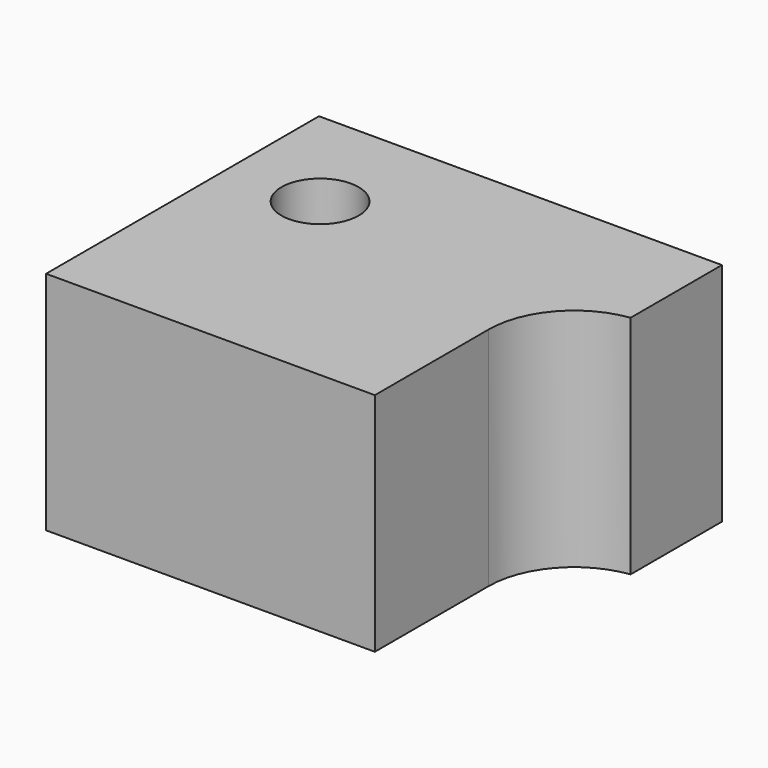
from build123d import *

# Parameters (mm, degrees)
F0_W        = 909.2783331871
F0_H        = 769.7594761848
F0_R        = 87.1640503321
F1_DEPTH    = 509.82533
F2_W        = 512.1824108064
F2_H        = 509.82533
F3_DEPTH    = 167.38894
F4_T1_DEPTH = 509.82533


# Not quite as in the source:
# - a fillet or chamfer that OpenCascade refuses, or shapes differently, is made with other operations: its cross-section is extruded or revolved along the edge and cut away or added


with BuildPart() as f1:
    # F0 (on Top) → F1 (new body)
    with BuildSketch(Plane.XY):
        with Locations((-191.2371218204, -78.1787037849)):
            Rectangle(F0_W, F0_H)
        with Locations((-441.408932209, 54.1237108409)):
            Circle(F0_R, mode=Mode.SUBTRACT)
    extrude(amount=F1_DEPTH)

    # F2 (on face) → F3 (cut)
    with BuildSketch(Plane.YZ.offset(263.4020447731)):
        with Locations((-206.9672364742, 254.912665)):
            Rectangle(F2_W, F2_H)
    extrude(amount=-F3_DEPTH, mode=Mode.SUBTRACT)

    # F4: fillet of radius 192.8795849713 on 1 edges, made by hand

    # F4_s2 → F4_t1 (join)
    with BuildSketch(Plane.XY):
        with BuildLine():
            ThreePointArc((263.4020447731, 49.1239689291), (143.7734985232, -15.0088679899), (96.0131047731, -142.0637956315))
            Line((96.0131047731, -142.0637956315), (96.0131047731, 49.1239689291))
            Line((96.0131047731, 49.1239689291), (263.4020447731, 49.1239689291))
        make_face()
    extrude(amount=F4_T1_DEPTH)


solid = f1.part
